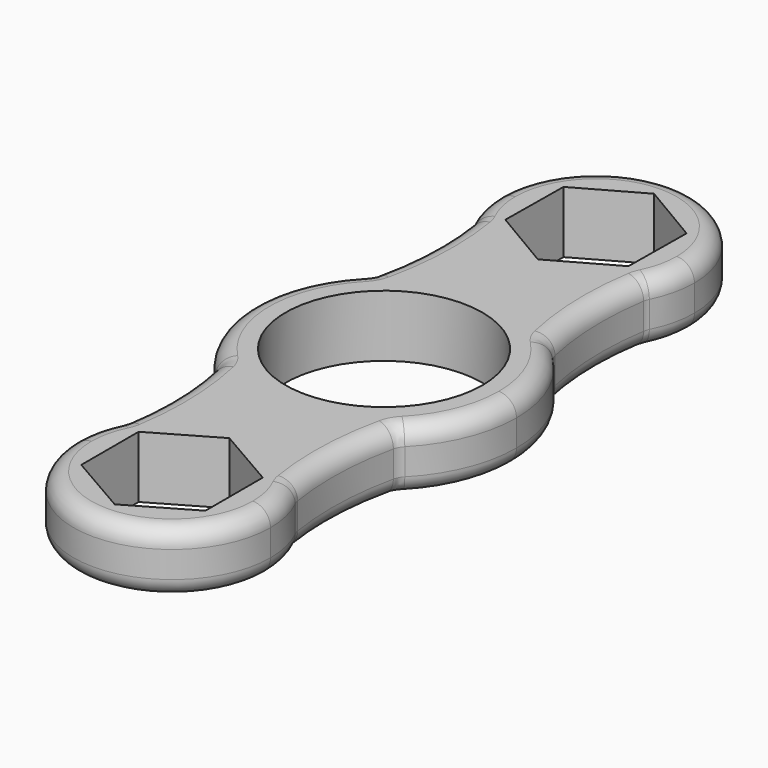
from build123d import *

# Parameters (mm, degrees)
F0_R     = 11.15
F1_DEPTH = 7
F2_F1_R  = 2
F2_F2_R  = 2


with BuildPart() as f1:
    # F0 (on Top) → F1 (new body)
    with BuildSketch(Plane.XY):
        with BuildLine():
            ThreePointArc((9.8633666231, 24.8003366592), (10.4070661449, 27.4248181508), (11.15, 30))
            ThreePointArc((11.15, 30), (0, 41.15), (-11.15, 30))
            ThreePointArc((-11.15, 30), (-10.4070661449, 27.4248181508), (-9.8633666231, 24.8003366592))
            ThreePointArc((-9.8633666231, 24.8003366592), (0, 18.85), (9.8633666231, 24.8003366592))
        make_face()
        Polygon((7.071897316, 33.9815853102), (6.984102684, 25.8663499265), (-0.087794632, 21.8847646163), (-7.071897316, 26.0184146898), (-6.984102684, 34.1336500735), (0.087794632, 38.1152353837), align=None, mode=Mode.SUBTRACT)
        with BuildLine():
            ThreePointArc((9.8633666231, 24.8003366592), (10.8235631344, 27.3217578384), (11.15, 30))
            ThreePointArc((11.15, 30), (10.4070661449, 27.4248181508), (9.8633666231, 24.8003366592))
        make_face()
        with BuildLine():
            ThreePointArc((-9.8633666231, 24.8003366592), (-10.4070661449, 27.4248181508), (-11.15, 30))
            ThreePointArc((-11.15, 30), (-10.8235631344, 27.3217578384), (-9.8633666231, 24.8003366592))
        make_face()
        with BuildLine():
            ThreePointArc((10.3461667366, 10.8607934267), (9.4033506208, 17.8062712948), (9.8633666231, 24.8003366592))
            ThreePointArc((9.8633666231, 24.8003366592), (0, 18.85), (-9.8633666231, 24.8003366592))
            ThreePointArc((-9.8633666231, 24.8003366592), (-9.4033506208, 17.8062712948), (-10.3461667366, 10.8607934267))
            ThreePointArc((-10.3461667366, 10.8607934267), (0, 15), (10.3461667366, 10.8607934267))
        make_face()
        with BuildLine():
            ThreePointArc((15, 0), (13.7875396835, 5.9079395288), (10.3461667366, 10.8607934267))
            ThreePointArc((10.3461667366, 10.8607934267), (0, 15), (-10.3461667366, 10.8607934267))
            ThreePointArc((-10.3461667366, 10.8607934267), (-15, 0), (-10.3461667366, -10.8607934267))
            ThreePointArc((-10.3461667366, -10.8607934267), (0, -15), (10.3461667366, -10.8607934267))
            ThreePointArc((10.3461667366, -10.8607934267), (13.7875396835, -5.9079395288), (15, 0))
        make_face()
        Circle(F0_R, mode=Mode.SUBTRACT)
        with BuildLine():
            ThreePointArc((10.3461667366, -10.8607934267), (0, -15), (-10.3461667366, -10.8607934267))
            ThreePointArc((-10.3461667366, -10.8607934267), (-9.4033506208, -17.8062712948), (-9.8633666231, -24.8003366592))
            ThreePointArc((-9.8633666231, -24.8003366592), (0, -18.85), (9.8633666231, -24.8003366592))
            ThreePointArc((9.8633666231, -24.8003366592), (9.4033506208, -17.8062712948), (10.3461667366, -10.8607934267))
        make_face()
        with BuildLine():
            ThreePointArc((-11.15, -30), (-10.4070661449, -27.4248181508), (-9.8633666231, -24.8003366592))
            ThreePointArc((-9.8633666231, -24.8003366592), (-10.8235631344, -27.3217578384), (-11.15, -30))
        make_face()
        with BuildLine():
            ThreePointArc((9.8633666231, -24.8003366592), (0, -18.85), (-9.8633666231, -24.8003366592))
            ThreePointArc((-9.8633666231, -24.8003366592), (-10.4070661449, -27.4248181508), (-11.15, -30))
            ThreePointArc((-11.15, -30), (0, -41.15), (11.15, -30))
            ThreePointArc((11.15, -30), (10.4070661449, -27.4248181508), (9.8633666231, -24.8003366592))
        make_face()
        Polygon((0, -38.1152353837), (-7.028, -34.0576176919), (-7.028, -25.9423823081), (0, -21.8847646163), (7.028, -25.9423823081), (7.028, -34.0576176919), align=None, mode=Mode.SUBTRACT)
        with BuildLine():
            ThreePointArc((11.15, -30), (10.8235631344, -27.3217578384), (9.8633666231, -24.8003366592))
            ThreePointArc((9.8633666231, -24.8003366592), (10.4070661449, -27.4248181508), (11.15, -30))
        make_face()
    extrude(amount=F1_DEPTH)

    # F2: fillet of radius 2 on 16 edges, made by hand

    # F2_f1
    f2_f1_edges = [f1.edges().sort_by_distance(p)[0] for p in [
        (9.8633666231, 24.8003366592, 3.5),
        (-9.8633666231, 24.8003366592, 3.5),
        (-10.3461667366, 10.8607934267, 3.5),
        (-10.3461667366, -10.8607934267, 3.5),
        (-9.8633666231, -24.8003366592, 3.5),
        (9.8633666231, -24.8003366592, 3.5),
        (10.3461667366, -10.8607934267, 3.5),
        (10.3461667366, 10.8607934267, 3.5),
    ]]
    fillet(f2_f1_edges, radius=F2_F1_R)

    # F2_f2
    f2_f2_edges = [f1.edges().sort_by_distance(p)[0] for p in [
        (0, 41.15, 0),
        (0, 41.15, 7),
        (-15, 0, 0),
        (-15, 0, 7),
        (0, -41.15, 0),
        (0, -41.15, 7),
        (15, 0, 0),
        (15, 0, 7),
        (10.4053953585, -10.9238749782, 7),
        (10.4053953585, 10.9238749782, 7),
        (10.4053953585, -10.9238749782, 0),
        (10.4053953585, 10.9238749782, 0),
        (-9.8812276283, -24.7765420656, 7),
        (9.8812276283, -24.7765420656, 7),
        (-9.8812276283, -24.7765420656, 0),
        (9.8812276283, -24.7765420656, 0),
        (-10.4053953585, 10.9238749782, 7),
        (-10.4053953585, -10.9238749782, 7),
        (-10.4053953585, 10.9238749782, 0),
        (-10.4053953585, -10.9238749782, 0),
        (9.8812276283, 24.7765420656, 7),
        (-9.8812276283, 24.7765420656, 7),
        (9.8812276283, 24.7765420656, 0),
        (-9.8812276283, 24.7765420656, 0),
    ]]
    fillet(f2_f2_edges, radius=F2_F2_R)


solid = f1.part
